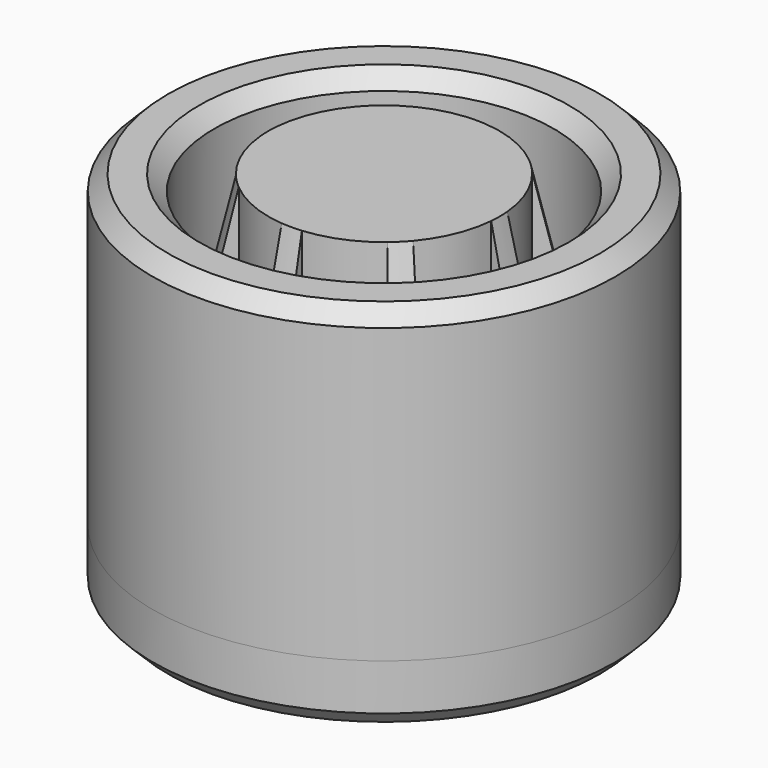
from build123d import *

# Parameters (mm, degrees)
F0_R            = 15
F0_R_2          = 11
F0_R_3          = 7.5
F1_DEPTH        = 4
F2_DEPTH        = 20
F4_ANGLE_BACK   = 5
F4_ANGLE        = 10
F4_COPIES_COUNT = 8
F5_SIZE         = 1


# Not quite as in the source:
# - a pattern or mirror of a feature is missing from the dataset's text; its kind, count and spacing are read off the source's solid


with BuildPart() as f1:
    # F0 (on Top) → F1 (new body)
    with BuildSketch(Plane.XY):
        Circle(F0_R)
        Circle(F0_R_2, mode=Mode.SUBTRACT)
        Circle(F0_R_2)
        Circle(F0_R_3, mode=Mode.SUBTRACT)
        Circle(F0_R_3)
    extrude(amount=-F1_DEPTH)

    # F0 (on Top) → F2 (join)
    with BuildSketch(Plane.XY):
        Circle(F0_R)
        Circle(F0_R_2, mode=Mode.SUBTRACT)
        Circle(F0_R_3)
    extrude(amount=F2_DEPTH)

    # F3 (on Front) → F4 (revolve)
    with BuildSketch(Plane.XZ, mode=Mode.PRIVATE) as f4_sk:
        Polygon((0, 20), (0, 0), (7.5, 0), (10.3, 8), (7.5, 20), align=None)
    f4 = revolve(f4_sk.sketch.rotate(Axis((0, 0, 10), (0, 0, 1)), -F4_ANGLE_BACK), axis=Axis((0, 0, 10), (0, 0, 1)), revolution_arc=F4_ANGLE)

    # F4_copies: F4 ×8 about axis
    f4_copies_axis = Axis((0, 0, 0), (0, 0, 1))
    for i in range(1, F4_COPIES_COUNT):
        add(f4.rotate(f4_copies_axis, i * 360 / F4_COPIES_COUNT))

    # F5
    f5_edges = [f1.edges().sort_by_distance(p)[0] for p in [
        (-15, 0, 20),
        (-11, 0, 20),
        (-15, 0, -4),
    ]]
    chamfer(f5_edges, length=F5_SIZE)


solid = f1.part
